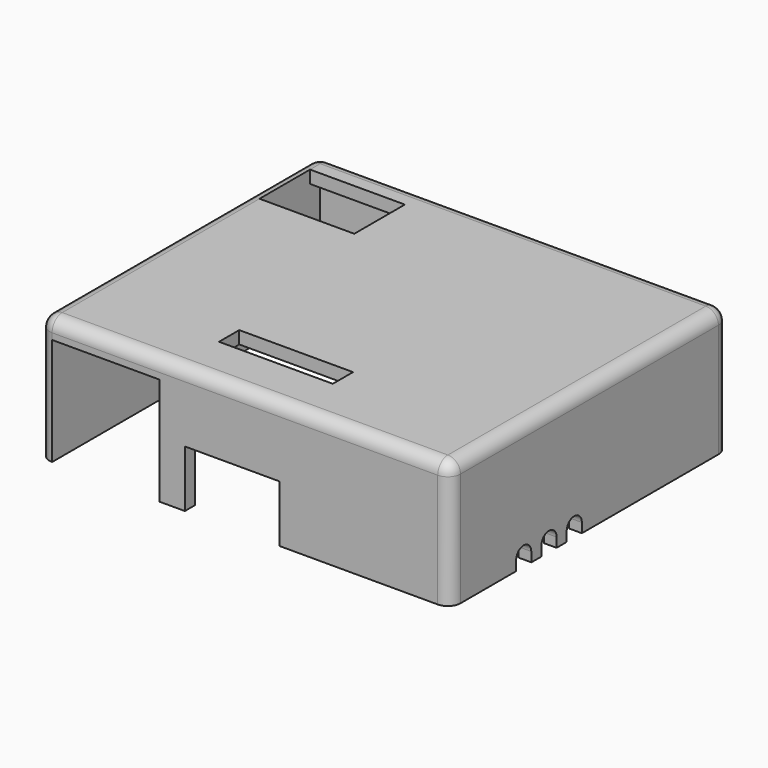
from build123d import *

# Parameters (mm, degrees)
F0_W     = 65
F0_H     = 55
F1_DEPTH = 10
F2_T     = -2
F3_W     = 17
F3_H     = 17
F3_W_2   = 15
F3_H_2   = 9
F4_DEPTH = 27.5
F6_DEPTH = 25.4
F7_W     = 15
F7_H     = 10
F7_W_2   = 18
F7_H_2   = 4
F8_DEPTH = 12.7
F9_R     = 1.99999


# Not quite as in the source:
# - a fillet or chamfer is up to 0.001 mm smaller than in the source, because OpenCascade refuses the exact size


with BuildPart() as f1:
    # F0 (on Top) → F1 (new body, symmetric)
    with BuildSketch(Plane.XY):
        Rectangle(F0_W, F0_H)
    extrude(amount=F1_DEPTH, both=True)

    # F2
    f2_openings = [f1.faces().sort_by_distance(p)[0] for p in [
        (0, 0, -10),
    ]]
    offset(amount=F2_T, openings=f2_openings)

    # F3 (on Front) → F4 (cut, through all)
    with BuildSketch(Plane.XZ):
        with Locations((-22, -1.5)):
            Rectangle(F3_W, F3_H)
        with Locations((-2, -5.5)):
            Rectangle(F3_W_2, F3_H_2)
    extrude(amount=F4_DEPTH, mode=Mode.SUBTRACT)

    # F5 (on face) → F6 (cut)
    with BuildSketch(Plane.YZ.offset(32.5)):
        with BuildLine():
            Line((-14.5, -10), (-13, -10))
            ThreePointArc((-13, -10), (-14.0606601718, -9.5606601718), (-14.5, -8.5))
            Line((-14.5, -8.5), (-14.5, -10))
        make_face()
        with BuildLine():
            ThreePointArc((-13, -10), (-11.9393398282, -9.5606601718), (-11.5, -8.5))
            ThreePointArc((-11.5, -8.5), (-11.5000361058, -8.4895924938), (-11.5001444216, -8.4791854886))
            ThreePointArc((-11.5001444216, -8.4791854886), (-13.0104075062, -7.0000361058), (-14.5, -8.5))
            ThreePointArc((-14.5, -8.5), (-14.0606601718, -9.5606601718), (-13, -10))
        make_face()
        with BuildLine():
            ThreePointArc((-11.5001444216, -8.4791854886), (-11.5000361058, -8.4895924938), (-11.5, -8.5))
            ThreePointArc((-11.5, -8.5), (-11.9393398282, -9.5606601718), (-13, -10))
            Line((-13, -10), (-11.4790390489, -10))
            Line((-11.4790390489, -10), (-11.5001444216, -8.4791854886))
        make_face()
        with BuildLine():
            ThreePointArc((-6.5, -8.5), (-8, -7), (-9.5, -8.5))
            ThreePointArc((-9.5, -8.5), (-9.0606601747, -9.5606601688), (-8.0000000084, -10))
            ThreePointArc((-8.0000000084, -10), (-6.9393398312, -9.5606601747), (-6.5, -8.5))
        make_face()
        with BuildLine():
            Line((-9.5, -8.5), (-9.5, -10))
            Line((-9.5, -10), (-8.0000000084, -10))
            ThreePointArc((-8.0000000084, -10), (-9.0606601747, -9.5606601688), (-9.5, -8.5))
        make_face()
        with BuildLine():
            ThreePointArc((-6.5, -8.5), (-6.9393398312, -9.5606601747), (-8.0000000084, -10))
            Line((-8.0000000084, -10), (-6.5, -10))
            Line((-6.5, -10), (-6.5, -8.5))
        make_face()
        with BuildLine():
            ThreePointArc((-1.5, -8.5), (-3, -7), (-4.5, -8.5))
            ThreePointArc((-4.5, -8.5), (-4.0606601718, -9.5606601718), (-3, -10))
            ThreePointArc((-3, -10), (-1.9393398282, -9.5606601718), (-1.5, -8.5))
        make_face()
        with BuildLine():
            Line((-4.5, -8.5), (-4.5, -10))
            Line((-4.5, -10), (-3, -10))
            ThreePointArc((-3, -10), (-4.0606601718, -9.5606601718), (-4.5, -8.5))
        make_face()
        with BuildLine():
            ThreePointArc((-1.5, -8.5), (-1.9393398282, -9.5606601718), (-3, -10))
            Line((-3, -10), (-1.5, -10))
            Line((-1.5, -10), (-1.5, -8.5))
        make_face()
    extrude(amount=-F6_DEPTH, mode=Mode.SUBTRACT)

    # F7 (on face) → F8 (cut, symmetric)
    with BuildSketch(Plane.XY.offset(10)):
        with Locations((-23, 18.5)):
            Rectangle(F7_W, F7_H)
        with Locations((-1.5, -17.5)):
            Rectangle(F7_W_2, F7_H_2)
    extrude(amount=F8_DEPTH, both=True, mode=Mode.SUBTRACT)

    # F9 (radius 2 in the source; OpenCascade refuses exactly that, so slightly less here)
    f9_edges = [f1.edges().sort_by_distance(p)[0] for p in [
        (-32.5, -27.5, 0),
        (32.5, -27.5, 0),
        (32.5, 27.5, 0),
        (-32.5, 27.5, 0),
        (0, -27.5, 10),
        (32.5, 0, 10),
        (0, 27.5, 10),
        (-32.5, 0, 10),
    ]]
    fillet(f9_edges, radius=F9_R)


solid = f1.part
